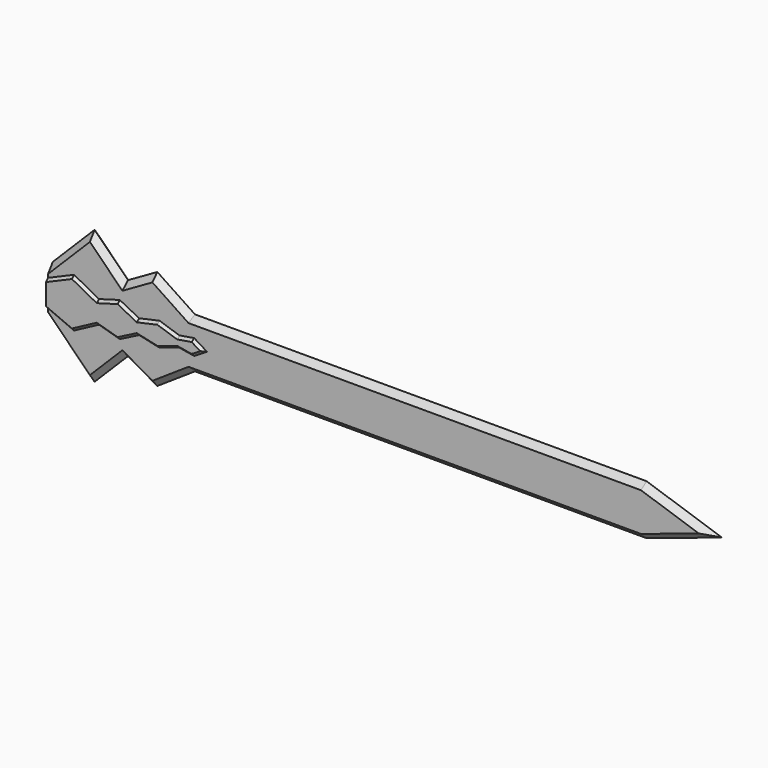
from build123d import *

# Parameters (mm, degrees)
F1_DEPTH = 7
F2_SIZE  = 6.99999
F4_DEPTH = 3
F5_SIZE  = 2.99999


# Not quite as in the source:
# - a fillet or chamfer is up to 0.001 mm smaller than in the source, because OpenCascade refuses the exact size


with BuildPart() as f1:
    # F0 (on Front) → F1 (new body)
    with BuildSketch(Plane.XZ):
        Polygon((0, 30), (0, 0), (800, 0), (710, 30), (170, 30), (125, 60), (90, 40), (50, 80), align=None)
        Polygon((800, 0), (0, 0), (0, -30), (50, -80), (90, -40), (125, -60), (170, -30), (710, -30), align=None)
    extrude(amount=F1_DEPTH)

    # F2 (size 7 in the source; OpenCascade refuses exactly that, so slightly less here)
    f2_edges = [f1.edges().sort_by_distance(p)[0] for p in [
        (25, -7, 55),
        (70, -7, 60),
        (107.5, -7, 50),
        (147.5, -7, 45),
        (440, -7, 30),
        (755, -7, 15),
        (25, -7, -55),
        (70, -7, -60),
        (107.5, -7, -50),
        (147.5, -7, -45),
        (440, -7, -30),
        (755, -7, -15),
    ]]
    chamfer(f2_edges, length=F2_SIZE)

    # F3 (on face) → F4 (join)
    with BuildSketch(Plane.XZ.offset(7)):
        Polygon((173.4544423223, -3.2363315113), (190, 0), (0, 0), (0, -16.0339120775), (30.4576978087, -14.7672765888), (60.9153956175, -13.5006411001), (84.8846249282, -11.1722019501), (108.853854239, -8.8437628001), (132.8813694417, -7.6582129113), (156.9088846445, -6.4726630226), align=None)
        Polygon((173.4544423223, 3.2363315113), (190, 0), (174.6631610562, 9.4158361321), align=None)
        Polygon((0, 0), (190, 0), (173.4544423223, 3.2363315113), (156.9088846445, 6.4726630226), (132.8813694417, 7.6582129113), (108.853854239, 8.8437628001), (84.8846249282, 11.1722019501), (60.9153956175, 13.5006411001), (30.4576978087, 14.7672765888), (0, 16.0339120775), align=None)
        Polygon((174.6631610562, -9.4158361321), (190, 0), (173.4544423223, -3.2363315113), align=None)
        Polygon((173.4544423223, 3.2363315113), (174.6631610562, 9.4158361321), (156.9088846445, 6.4726630226), align=None)
        Polygon((174.6631610562, -9.4158361321), (173.4544423223, -3.2363315113), (156.9088846445, -6.4726630226), align=None)
        Polygon((31.0645442111, 29.359591825), (0, 16.0339120775), (30.4576978087, 14.7672765888), align=None)
        Polygon((30.4576978087, -14.7672765888), (0, -16.0339120775), (31.0645442111, -29.359591825), align=None)
        Polygon((132.8813694417, 7.6582129113), (156.9088846445, 6.4726630226), (133.2047409049, 14.2119757014), align=None)
        Polygon((133.2047409049, -14.2119757014), (156.9088846445, -6.4726630226), (132.8813694417, -7.6582129113), align=None)
        Polygon((60.9153956175, 13.5006411001), (31.0645442111, 29.359591825), (30.4576978087, 14.7672765888), align=None)
        Polygon((30.4576978087, -14.7672765888), (31.0645442111, -29.359591825), (60.9153956175, -13.5006411001), align=None)
        Polygon((132.8813694417, 7.6582129113), (133.2047409049, 14.2119757014), (108.853854239, 8.8437628001), align=None)
        Polygon((108.853854239, -8.8437628001), (133.2047409049, -14.2119757014), (132.8813694417, -7.6582129113), align=None)
        Polygon((85.8007351026, 20.602748951), (60.9153956175, 13.5006411001), (84.8846249282, 11.1722019501), align=None)
        Polygon((84.8846249282, -11.1722019501), (60.9153956175, -13.5006411001), (85.8007351026, -20.602748951), align=None)
        Polygon((84.8846249282, 11.1722019501), (108.853854239, 8.8437628001), (85.8007351026, 20.602748951), align=None)
        Polygon((85.8007351026, -20.602748951), (108.853854239, -8.8437628001), (84.8846249282, -11.1722019501), align=None)
    extrude(amount=F4_DEPTH)

    # F5 (size 3 in the source; OpenCascade refuses exactly that, so slightly less here)
    f5_edges = [f1.edges().sort_by_distance(p)[0] for p in [
        (15.532272, -10, 22.696752),
        (45.98997, -10, 21.430116),
        (73.358065, -10, 17.051695),
        (97.327295, -10, 14.723256),
        (121.029298, -10, 11.527869),
        (145.056813, -10, 10.342319),
        (165.786023, -10, 7.94425),
        (182.331581, -10, 4.707918),
        (182.331581, -10, -4.707918),
        (165.786023, -10, -7.94425),
        (145.056813, -10, -10.342319),
        (121.029298, -10, -11.527869),
        (97.327295, -10, -14.723256),
        (73.358065, -10, -17.051695),
        (45.98997, -10, -21.430116),
        (15.532272, -10, -22.696752),
    ]]
    chamfer(f5_edges, length=F5_SIZE)

    # F6: F1 across plane


with BuildPart() as f1_1:
    add(f1.part)
    add(f1.part.mirror(Plane.XZ))


solid = f1_1.part
